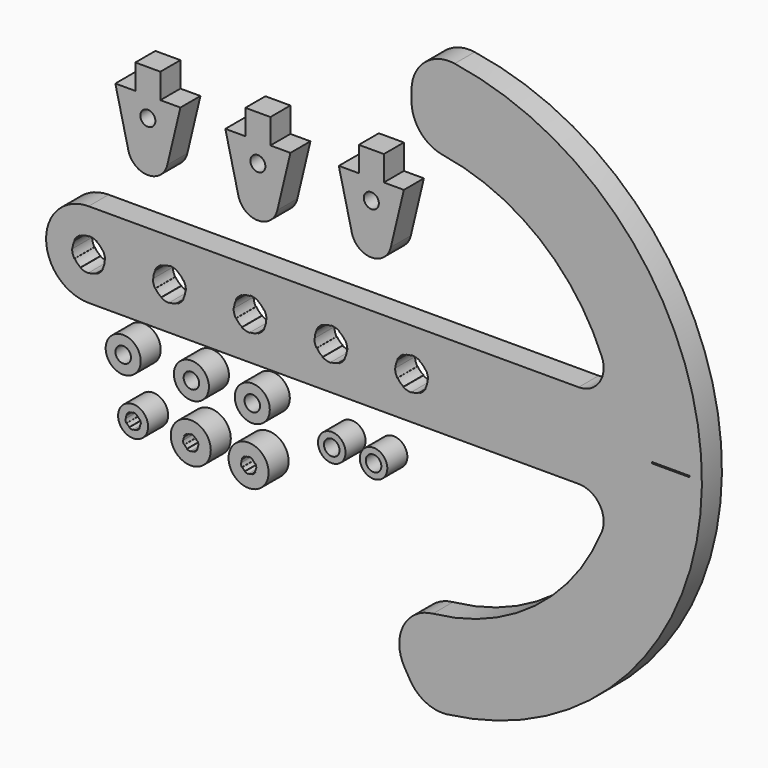
from build123d import *

# Parameters (mm, degrees)
F0_R     = 3
F1_DEPTH = 10
F0_R_2   = 6
F0_W     = 15
F0_H     = 0.5
F0_R_3   = 8
F0_R_4   = 5.5
F0_R_5   = 3.1
F0_R_6   = 7


# Not quite as in the source:
# - ends of sketch curves that miss each other by under 0.0002 mm in the source are joined


with BuildPart() as f1:
    # F0 (on Front) → F1 (new body)
    with BuildSketch(Plane.XZ):
        with BuildLine():
            Line((-95.3376, 63.814411), (-103.3376, 63.814411))
            Line((-103.3376, 63.814411), (-98.118888, 41.956574))
            ThreePointArc((-98.1188879236, 41.9565740183), (-90.3376, 35.814411), (-82.5563120764, 41.9565740183))
            Line((-82.556312, 41.956574), (-77.3376, 63.814411))
            Line((-77.3376, 63.814411), (-85.3376, 63.814411))
            Line((-85.3376, 63.814411), (-85.3376, 73.814411))
            Line((-85.3376, 73.814411), (-95.3376, 73.814411))
            Line((-95.3376, 73.814411), (-95.3376, 63.814411))
        make_face()
        with Locations((-90.3376, 55.814411)):
            Circle(F0_R, mode=Mode.SUBTRACT)
    extrude(amount=F1_DEPTH)


with BuildPart() as f1b:
    # F0 (on Front) → F1, piece 2 (new body)
    with BuildSketch(Plane.XZ):
        with BuildLine():
            Line((-51.390768, 62.163825), (-59.390768, 62.163825))
            Line((-59.390768, 62.163825), (-54.172056, 40.305987))
            ThreePointArc((-54.172056, 40.305987), (-46.390768, 34.163825), (-38.6094803023, 40.3059870722))
            Line((-38.6094803023, 40.3059870722), (-33.390768, 62.163825))
            Line((-33.390768, 62.163825), (-41.390768, 62.163825))
            Line((-41.390768, 62.163825), (-41.390768, 72.163825))
            Line((-41.390768, 72.163825), (-51.390768, 72.163825))
            Line((-51.390768, 72.163825), (-51.390768, 62.163825))
        make_face()
        with Locations((-46.390768, 54.163825)):
            Circle(F0_R, mode=Mode.SUBTRACT)
    extrude(amount=F1_DEPTH)


with BuildPart() as f1c:
    # F0 (on Front) → F1, piece 3 (new body)
    with BuildSketch(Plane.XZ):
        with BuildLine():
            Line((3.934353, 73.887845), (-6.065647, 73.887845))
            Line((-6.065647, 73.887845), (-6.065647, 63.887845))
            Line((-6.065647, 63.887845), (-14.065647, 63.887845))
            Line((-14.065647, 63.887845), (-8.846935, 42.030008))
            ThreePointArc((-8.8469349236, 42.0300080183), (-1.065647, 35.887845), (6.7156409236, 42.0300080183))
            Line((6.715641, 42.030008), (11.934353, 63.887845))
            Line((11.934353, 63.887845), (3.934353, 63.887845))
            Line((3.934353, 63.887845), (3.934353, 73.887845))
        make_face()
        with Locations((-1.065647, 55.887845)):
            Circle(F0_R, mode=Mode.SUBTRACT)
    extrude(amount=F1_DEPTH)


with BuildPart() as f1d:
    # F0 (on Front) → F1, piece 4 (new body)
    with BuildSketch(Plane.XZ):
        with Locations((-96.238976, -52.650425)):
            Circle(F0_R_2)
        with BuildLine():
            ThreePointArc((-93.5542974362, -54.2004253255), (-94.0469451551, -54.8424561985), (-94.6889761075, -55.3351038138))
            Line((-94.6889761075, -55.3351038138), (-94.788976, -55.161899))
            ThreePointArc((-94.788976, -55.161899), (-95.4884008487, -55.4516099175), (-96.238976, -55.550425))
            Line((-96.238976, -55.550425), (-96.238976, -55.750425))
            ThreePointArc((-96.238976, -55.750425), (-97.0413149799, -55.6447950776), (-97.7889758925, -55.3351038138))
            Line((-97.7889758925, -55.3351038138), (-97.688976, -55.161899))
            ThreePointArc((-97.688976, -55.161899), (-98.2895856654, -54.7010346654), (-98.7504497532, -54.1004248575))
            Line((-98.7504497532, -54.1004248575), (-98.923655, -54.200425))
            ThreePointArc((-98.923655, -54.200425), (-99.2333460776, -53.4527639799), (-99.338976, -52.650425))
            Line((-99.338976, -52.650425), (-99.138976, -52.650425))
            ThreePointArc((-99.138976, -52.650425), (-99.0401609175, -51.8998498487), (-98.7504497532, -51.2004251425))
            Line((-98.7504497532, -51.2004251425), (-98.923655, -51.100425))
            ThreePointArc((-98.923655, -51.100425), (-98.4310071985, -50.4583941551), (-97.7889763255, -49.9657464362))
            Line((-97.7889763255, -49.9657464362), (-97.688976, -50.138952))
            ThreePointArc((-97.688976, -50.138952), (-96.9895513928, -49.8492401472), (-96.238976, -49.750425))
            Line((-96.238976, -49.750425), (-96.238976, -49.550425))
            ThreePointArc((-96.238976, -49.550425), (-95.4366367787, -49.6560549871), (-94.6889756745, -49.9657464362))
            Line((-94.6889756745, -49.9657464362), (-94.788976, -50.138952))
            ThreePointArc((-94.788976, -50.138952), (-94.1883663346, -50.5998153346), (-93.7275024968, -51.2004247095))
            Line((-93.7275024968, -51.2004247095), (-93.554298, -51.100425))
            ThreePointArc((-93.554298, -51.100425), (-93.2446059871, -51.8480857787), (-93.138976, -52.650425))
            Line((-93.138976, -52.650425), (-93.338976, -52.650425))
            ThreePointArc((-93.338976, -52.650425), (-93.4377911472, -53.4010003928), (-93.7275024968, -54.1004252905))
            Line((-93.7275024968, -54.1004252905), (-93.5542974362, -54.2004253255))
        make_face(mode=Mode.SUBTRACT)
    extrude(amount=F1_DEPTH)


with BuildPart() as f1e:
    # F0 (on Front) → F1, piece 5 (new body)
    with BuildSketch(Plane.XZ):
        with BuildLine():
            Line((81.745787, 17.183144), (-114, 17.183144))
            ThreePointArc((-114, 17.183144), (-131, 0.183144), (-114, -16.816856))
            Line((-114, -16.816856), (81.745787, -16.816856))
            ThreePointArc((81.745787, -16.816856), (90.0373489873, -21.2266860732), (91.0160350936, -30.5668560378))
            ThreePointArc((91.0160350936, -30.5668560378), (64.3230219839, -65.3244090178), (23.5416670094, -81.3707640897))
            ThreePointArc((23.5416670094, -81.3707640897), (11.7178159843, -89.5211770694), (12.1637574003, -103.8750557654))
            Line((12.1637574003, -103.8750557654), (14.376089, -107.648966))
            ThreePointArc((14.376089, -107.648966), (20.6685505139, -113.50943883), (29.1456819886, -114.9511239073))
            ThreePointArc((29.1456819886, -114.9511239073), (130.9895728565, -1.3721657959), (32.2277229324, 114.8967245498))
            ThreePointArc((32.2277229324, 114.8967245498), (20.2126572599, 111.4300382658), (15, 100.063072))
            Line((15, 100.063072), (15, 96.016333))
            ThreePointArc((15, 96.016333), (18.6027677543, 86.2642513177), (27.6804129518, 81.1967676917))
            ThreePointArc((27.6804129518, 81.1967676917), (65.9742376399, 64.4141886516), (91.0160345641, 30.9331438237))
            ThreePointArc((91.0160345641, 30.9331438237), (90.0373489873, 21.5929740732), (81.745787, 17.183144))
        make_face()
        with BuildLine():
            ThreePointArc((-120.4, 0.183144), (-120.1819252504, 1.8395860297), (-119.5425624382, 3.383144253))
            Line((-119.5425624382, 3.383144253), (-119.715767, 3.483144))
            ThreePointArc((-119.715767, 3.483144), (-118.6669045791, 4.8500489326), (-117.2999998549, 5.8989117487))
            Line((-117.2999998549, 5.8989117487), (-117.2, 5.725707))
            ThreePointArc((-117.2, 5.725707), (-115.6564417883, 6.3650693152), (-114, 6.583144))
            Line((-114, 6.583144), (-114, 6.783144))
            ThreePointArc((-114, 6.783144), (-112.2917943832, 6.5582544752), (-110.7000001451, 5.8989117487))
            Line((-110.7000001451, 5.8989117487), (-110.8, 5.725707))
            ThreePointArc((-110.8, 5.725707), (-109.4745166004, 4.7086273996), (-108.4574373118, 3.38314382))
            Line((-108.4574373118, 3.38314382), (-108.284232, 3.483144))
            ThreePointArc((-108.284232, 3.483144), (-107.6248895248, 1.8913496168), (-107.4, 0.183144))
            Line((-107.4, 0.183144), (-107.6, 0.183144))
            ThreePointArc((-107.6, 0.183144), (-107.8180746848, -1.4732977883), (-108.4574373118, -3.01685582))
            Line((-108.4574373118, -3.01685582), (-108.284232, -3.116856))
            ThreePointArc((-108.284232, -3.116856), (-109.3330950674, -4.4837605791), (-110.6999997121, -5.5326234987))
            Line((-110.6999997121, -5.5326234987), (-110.8, -5.359418))
            ThreePointArc((-110.8, -5.359418), (-112.3435579703, -5.9987812504), (-114, -6.216856))
            Line((-114, -6.216856), (-114, -6.416856))
            ThreePointArc((-114, -6.416856), (-115.7082058583, -6.1919664105), (-117.3000002879, -5.5326234987))
            Line((-117.3000002879, -5.5326234987), (-117.2, -5.359418))
            ThreePointArc((-117.2, -5.359418), (-118.5254833996, -4.3423393996), (-119.5425624382, -3.016856253))
            Line((-119.5425624382, -3.016856253), (-119.715767, -3.116856))
            ThreePointArc((-119.715767, -3.116856), (-120.3751104105, -1.5250618583), (-120.6, 0.183144))
            Line((-120.6, 0.183144), (-120.4, 0.183144))
        make_face(mode=Mode.SUBTRACT)
        with BuildLine():
            ThreePointArc((-87.4657674987, 3.4831442879), (-86.4169045791, 4.8500489326), (-85.0499998549, 5.8989117487))
            Line((-85.0499998549, 5.8989117487), (-84.95, 5.725707))
            ThreePointArc((-84.95, 5.725707), (-83.4064417883, 6.3650693152), (-81.75, 6.583144))
            Line((-81.75, 6.583144), (-81.75, 6.783144))
            ThreePointArc((-81.75, 6.783144), (-80.0417943832, 6.5582544752), (-78.4500001451, 5.8989117487))
            Line((-78.4500001451, 5.8989117487), (-78.55, 5.725707))
            ThreePointArc((-78.55, 5.725707), (-77.2245166004, 4.7086273996), (-76.2074373118, 3.38314382))
            Line((-76.2074373118, 3.38314382), (-76.034232, 3.483144))
            ThreePointArc((-76.034232, 3.483144), (-75.3748895248, 1.8913496168), (-75.15, 0.183144))
            Line((-75.15, 0.183144), (-75.35, 0.183144))
            ThreePointArc((-75.35, 0.183144), (-75.5680746848, -1.4732977883), (-76.2074373118, -3.01685582))
            Line((-76.2074373118, -3.01685582), (-76.034232, -3.116856))
            ThreePointArc((-76.034232, -3.116856), (-77.0830950674, -4.4837605791), (-78.4499997121, -5.5326234987))
            Line((-78.4499997121, -5.5326234987), (-78.55, -5.359418))
            ThreePointArc((-78.55, -5.359418), (-80.0935579703, -5.9987812504), (-81.75, -6.216856))
            Line((-81.75, -6.216856), (-81.75, -6.416856))
            ThreePointArc((-81.75, -6.416856), (-83.4582058583, -6.1919664105), (-85.0500002879, -5.5326234987))
            Line((-85.0500002879, -5.5326234987), (-84.95, -5.359418))
            ThreePointArc((-84.95, -5.359418), (-86.2754833996, -4.3423393996), (-87.2925624382, -3.016856253))
            Line((-87.2925624382, -3.016856253), (-87.465767, -3.116856))
            ThreePointArc((-87.465767, -3.116856), (-88.1251104105, -1.5250618583), (-88.35, 0.183144))
            Line((-88.35, 0.183144), (-88.15, 0.183144))
            ThreePointArc((-88.15, 0.183144), (-87.9319252504, 1.8395860297), (-87.2925624382, 3.383144253))
            Line((-87.2925624382, 3.383144253), (-87.4657674987, 3.4831442879))
        make_face(mode=Mode.SUBTRACT)
        with BuildLine():
            ThreePointArc((-55.2157674987, 3.4831442879), (-54.1669045791, 4.8500489326), (-52.7999998549, 5.8989117487))
            Line((-52.7999998549, 5.8989117487), (-52.7, 5.725707))
            ThreePointArc((-52.7, 5.725707), (-51.1564417883, 6.3650693152), (-49.5, 6.583144))
            Line((-49.5, 6.583144), (-49.5, 6.783144))
            ThreePointArc((-49.5, 6.783144), (-47.7917943832, 6.5582544752), (-46.2000001451, 5.8989117487))
            Line((-46.2000001451, 5.8989117487), (-46.3, 5.725707))
            ThreePointArc((-46.3, 5.725707), (-44.9745166004, 4.7086273996), (-43.9574373118, 3.38314382))
            Line((-43.9574373118, 3.38314382), (-43.784232, 3.483144))
            ThreePointArc((-43.784232, 3.483144), (-43.1248895248, 1.8913496168), (-42.9, 0.183144))
            Line((-42.9, 0.183144), (-43.1, 0.183144))
            ThreePointArc((-43.1, 0.183144), (-43.3180746848, -1.4732977883), (-43.9574373118, -3.01685582))
            Line((-43.9574373118, -3.01685582), (-43.784232, -3.116856))
            ThreePointArc((-43.784232, -3.116856), (-44.8330950674, -4.4837605791), (-46.1999997121, -5.5326234987))
            Line((-46.1999997121, -5.5326234987), (-46.3, -5.359418))
            ThreePointArc((-46.3, -5.359418), (-47.8435579703, -5.9987812504), (-49.5, -6.216856))
            Line((-49.5, -6.216856), (-49.5, -6.416856))
            ThreePointArc((-49.5, -6.416856), (-51.2082058583, -6.1919664105), (-52.8000002879, -5.5326234987))
            Line((-52.8000002879, -5.5326234987), (-52.7, -5.359418))
            ThreePointArc((-52.7, -5.359418), (-54.0254833996, -4.3423393996), (-55.0425624382, -3.016856253))
            Line((-55.0425624382, -3.016856253), (-55.215767, -3.116856))
            ThreePointArc((-55.215767, -3.116856), (-55.8751104105, -1.5250618583), (-56.1, 0.183144))
            Line((-56.1, 0.183144), (-55.9, 0.183144))
            ThreePointArc((-55.9, 0.183144), (-55.6819252504, 1.8395860297), (-55.0425624382, 3.383144253))
            Line((-55.0425624382, 3.383144253), (-55.2157674987, 3.4831442879))
        make_face(mode=Mode.SUBTRACT)
        with BuildLine():
            ThreePointArc((-17.25, 6.783144), (-15.5417943832, 6.5582544752), (-13.9500001451, 5.8989117487))
            Line((-13.9500001451, 5.8989117487), (-14.05, 5.725707))
            ThreePointArc((-14.05, 5.725707), (-12.7245166004, 4.7086273996), (-11.7074373118, 3.38314382))
            Line((-11.7074373118, 3.38314382), (-11.534232, 3.483144))
            ThreePointArc((-11.534232, 3.483144), (-10.8748895248, 1.8913496168), (-10.65, 0.183144))
            Line((-10.65, 0.183144), (-10.85, 0.183144))
            ThreePointArc((-10.85, 0.183144), (-11.0680746848, -1.4732977883), (-11.7074373118, -3.01685582))
            Line((-11.7074373118, -3.01685582), (-11.534232, -3.116856))
            ThreePointArc((-11.534232, -3.116856), (-12.5830950674, -4.4837605791), (-13.9499997121, -5.5326234987))
            Line((-13.9499997121, -5.5326234987), (-14.05, -5.359418))
            ThreePointArc((-14.05, -5.359418), (-15.5935579703, -5.9987812504), (-17.25, -6.216856))
            Line((-17.25, -6.216856), (-17.25, -6.416856))
            ThreePointArc((-17.25, -6.416856), (-18.9582058583, -6.1919664105), (-20.5500002879, -5.5326234987))
            Line((-20.5500002879, -5.5326234987), (-20.45, -5.359418))
            ThreePointArc((-20.45, -5.359418), (-21.7754833996, -4.3423393996), (-22.7925624382, -3.016856253))
            Line((-22.7925624382, -3.016856253), (-22.965767, -3.116856))
            ThreePointArc((-22.965767, -3.116856), (-23.6251104105, -1.5250618583), (-23.85, 0.183144))
            Line((-23.85, 0.183144), (-23.65, 0.183144))
            ThreePointArc((-23.65, 0.183144), (-23.4319252504, 1.8395860297), (-22.7925624382, 3.383144253))
            Line((-22.7925624382, 3.383144253), (-22.965767, 3.483144))
            ThreePointArc((-22.965767, 3.483144), (-21.9169045791, 4.8500489326), (-20.5499998549, 5.8989117487))
            Line((-20.5499998549, 5.8989117487), (-20.45, 5.725707))
            ThreePointArc((-20.45, 5.725707), (-18.9064417883, 6.3650693152), (-17.25, 6.583144))
            Line((-17.25, 6.583144), (-17.25, 6.783144))
        make_face(mode=Mode.SUBTRACT)
        with BuildLine():
            ThreePointArc((15, 6.783144), (16.7082056168, 6.5582544752), (18.2999998549, 5.8989117487))
            Line((18.2999998549, 5.8989117487), (18.2, 5.725707))
            ThreePointArc((18.2, 5.725707), (19.5254833996, 4.7086273996), (20.5425626882, 3.38314382))
            Line((20.5425626882, 3.38314382), (20.715768, 3.483144))
            ThreePointArc((20.715768, 3.483144), (21.3751104752, 1.8913496168), (21.6, 0.183144))
            Line((21.6, 0.183144), (21.4, 0.183144))
            ThreePointArc((21.4, 0.183144), (21.1819253152, -1.4732977883), (20.5425626882, -3.01685582))
            Line((20.5425626882, -3.01685582), (20.715768, -3.116856))
            ThreePointArc((20.715768, -3.116856), (19.6669049326, -4.4837605791), (18.3000002879, -5.5326234987))
            Line((18.3000002879, -5.5326234987), (18.2, -5.359418))
            ThreePointArc((18.2, -5.359418), (16.6564420297, -5.9987812504), (15, -6.216856))
            Line((15, -6.216856), (15, -6.416856))
            ThreePointArc((15, -6.416856), (13.2917941417, -6.1919664105), (11.6999997121, -5.5326234987))
            Line((11.6999997121, -5.5326234987), (11.8, -5.359418))
            ThreePointArc((11.8, -5.359418), (10.4745166004, -4.3423393996), (9.4574375618, -3.016856253))
            Line((9.4574375618, -3.016856253), (9.284233, -3.116856))
            ThreePointArc((9.284233, -3.116856), (8.6248895895, -1.5250618583), (8.4, 0.183144))
            Line((8.4, 0.183144), (8.6, 0.183144))
            ThreePointArc((8.6, 0.183144), (8.8180747496, 1.8395860297), (9.4574375618, 3.383144253))
            Line((9.4574375618, 3.383144253), (9.284233, 3.483144))
            ThreePointArc((9.284233, 3.483144), (10.3330954209, 4.8500489326), (11.7000001451, 5.8989117487))
            Line((11.7000001451, 5.8989117487), (11.8, 5.725707))
            ThreePointArc((11.8, 5.725707), (13.3435582117, 6.3650693152), (15, 6.583144))
            Line((15, 6.583144), (15, 6.783144))
        make_face(mode=Mode.SUBTRACT)
        with Locations((118.5, 0.183144)):
            Rectangle(F0_W, F0_H, mode=Mode.SUBTRACT)
    extrude(amount=F1_DEPTH)


with BuildPart() as f1f:
    # F0 (on Front) → F1, piece 6 (new body)
    with BuildSketch(Plane.XZ):
        with Locations((-73.206252, -52.758697)):
            Circle(F0_R_3)
        with BuildLine():
            Line((-71.656252, -50.074018), (-71.756252, -50.247223))
            ThreePointArc((-71.756252, -50.247223), (-71.1556423346, -50.7080873346), (-70.6947782468, -51.3086971425))
            Line((-70.6947782468, -51.3086971425), (-70.521573, -51.208697))
            ThreePointArc((-70.521573, -51.208697), (-70.2118819224, -51.9563580201), (-70.106252, -52.758697))
            Line((-70.106252, -52.758697), (-70.306252, -52.758697))
            ThreePointArc((-70.306252, -52.758697), (-70.4050670825, -53.5092721513), (-70.6947782468, -54.2086968575))
            Line((-70.6947782468, -54.2086968575), (-70.521573, -54.308697))
            ThreePointArc((-70.521573, -54.308697), (-71.0142209783, -54.9507280217), (-71.6562521075, -55.4433758138))
            Line((-71.6562521075, -55.4433758138), (-71.756252, -55.270171))
            ThreePointArc((-71.756252, -55.270171), (-72.4556768487, -55.5598819175), (-73.206252, -55.658697))
            Line((-73.206252, -55.658697), (-73.206252, -55.858697))
            ThreePointArc((-73.206252, -55.858697), (-74.0085909799, -55.7530670776), (-74.7562518925, -55.4433758138))
            Line((-74.7562518925, -55.4433758138), (-74.656252, -55.270171))
            ThreePointArc((-74.656252, -55.270171), (-75.2568614887, -54.8093068422), (-75.7177255032, -54.2086972905))
            Line((-75.7177255032, -54.2086972905), (-75.89093, -54.308697))
            ThreePointArc((-75.89093, -54.308697), (-76.2006220129, -53.5610362213), (-76.306252, -52.758697))
            Line((-76.306252, -52.758697), (-76.106252, -52.758697))
            ThreePointArc((-76.106252, -52.758697), (-76.0074368528, -52.0081216072), (-75.7177255032, -51.3086967095))
            Line((-75.7177255032, -51.3086967095), (-75.89093, -51.208697))
            ThreePointArc((-75.89093, -51.208697), (-75.3982828449, -50.5666658015), (-74.7562518925, -50.0740181862))
            Line((-74.7562518925, -50.0740181862), (-74.656252, -50.247223))
            ThreePointArc((-74.656252, -50.247223), (-73.9568271513, -49.9575120825), (-73.206252, -49.858697))
            Line((-73.206252, -49.858697), (-73.206252, -49.658697))
            ThreePointArc((-73.206252, -49.658697), (-72.4039130201, -49.7643269224), (-71.656252, -50.074018))
        make_face(mode=Mode.SUBTRACT)
    extrude(amount=F1_DEPTH)


with BuildPart() as f1g:
    # F0 (on Front) → F1, piece 7 (new body)
    with BuildSketch(Plane.XZ):
        with Locations((-0.176901, -36.211649)):
            Circle(F0_R_4)
        with Locations((-0.176901, -36.211649)):
            Circle(F0_R_5, mode=Mode.SUBTRACT)
    extrude(amount=F1_DEPTH)


with BuildPart() as f1h:
    # F0 (on Front) → F1, piece 8 (new body)
    with BuildSketch(Plane.XZ):
        with Locations((-50.100666, -53.16348)):
            Circle(F0_R_3)
        with BuildLine():
            ThreePointArc((-52.7853448138, -51.6134801075), (-52.2926970217, -50.9714489783), (-51.6506658925, -50.4788011862))
            Line((-51.6506658925, -50.4788011862), (-51.550666, -50.652006))
            ThreePointArc((-51.550666, -50.652006), (-50.8512411513, -50.3622950825), (-50.100666, -50.26348))
            Line((-50.100666, -50.26348), (-50.100666, -50.06348))
            ThreePointArc((-50.100666, -50.06348), (-49.2983270201, -50.1691099224), (-48.5506661075, -50.4788011862))
            Line((-48.5506661075, -50.4788011862), (-48.650666, -50.652006))
            ThreePointArc((-48.650666, -50.652006), (-48.0500565113, -51.1128701578), (-47.5891924968, -51.7134797095))
            Line((-47.5891924968, -51.7134797095), (-47.415988, -51.61348))
            ThreePointArc((-47.415988, -51.61348), (-47.1062959871, -52.3611407787), (-47.000666, -53.16348))
            Line((-47.000666, -53.16348), (-47.200666, -53.16348))
            ThreePointArc((-47.200666, -53.16348), (-47.2994811472, -53.9140553928), (-47.5891924968, -54.6134802905))
            Line((-47.5891924968, -54.6134802905), (-47.415988, -54.71348))
            ThreePointArc((-47.415988, -54.71348), (-47.9086351551, -55.3555111985), (-48.5506661075, -55.8481588138))
            Line((-48.5506661075, -55.8481588138), (-48.650666, -55.674954))
            ThreePointArc((-48.650666, -55.674954), (-49.3500908487, -55.9646649175), (-50.100666, -56.06348))
            Line((-50.100666, -56.06348), (-50.100666, -56.26348))
            ThreePointArc((-50.100666, -56.26348), (-50.9030049799, -56.1578500776), (-51.6506658925, -55.8481588138))
            Line((-51.6506658925, -55.8481588138), (-51.550666, -55.674954))
            ThreePointArc((-51.550666, -55.674954), (-52.1512756654, -55.2140896654), (-52.6121397532, -54.6134798575))
            Line((-52.6121397532, -54.6134798575), (-52.785345, -54.71348))
            ThreePointArc((-52.785345, -54.71348), (-53.0950360776, -53.9658189799), (-53.200666, -53.16348))
            Line((-53.200666, -53.16348), (-53.000666, -53.16348))
            ThreePointArc((-53.000666, -53.16348), (-52.9018509175, -52.4129048487), (-52.6121397532, -51.7134801425))
            Line((-52.6121397532, -51.7134801425), (-52.7853448138, -51.6134801075))
        make_face(mode=Mode.SUBTRACT)
    extrude(amount=F1_DEPTH)


with BuildPart() as f1i:
    # F0 (on Front) → F1, piece 9 (new body)
    with BuildSketch(Plane.XZ):
        with Locations((-16.864495, -36.09547)):
            Circle(F0_R_4)
        with Locations((-16.864495, -36.09547)):
            Circle(F0_R_5, mode=Mode.SUBTRACT)
    extrude(amount=F1_DEPTH)


with BuildPart() as f1j:
    # F0 (on Front) → F1, piece 10 (new body)
    with BuildSketch(Plane.XZ):
        with Locations((-72.945373, -30.754178)):
            Circle(F0_R_6)
        with Locations((-72.945373, -30.754178)):
            Circle(F0_R_5, mode=Mode.SUBTRACT)
    extrude(amount=F1_DEPTH)


with BuildPart() as f1k:
    # F0 (on Front) → F1, piece 11 (new body)
    with BuildSketch(Plane.XZ):
        with Locations((-100.194918, -30.558139)):
            Circle(F0_R_6)
        with Locations((-100.194918, -30.558139)):
            Circle(F0_R_5, mode=Mode.SUBTRACT)
    extrude(amount=F1_DEPTH)


with BuildPart() as f1l:
    # F0 (on Front) → F1, piece 12 (new body)
    with BuildSketch(Plane.XZ):
        with Locations((-48.630373, -30.860699)):
            Circle(F0_R_6)
        with Locations((-48.630373, -30.860699)):
            Circle(F0_R_5, mode=Mode.SUBTRACT)
    extrude(amount=F1_DEPTH)


solid = Compound([f1.part, f1b.part, f1c.part, f1d.part, f1e.part, f1f.part, f1g.part, f1h.part, f1i.part, f1j.part, f1k.part, f1l.part])
